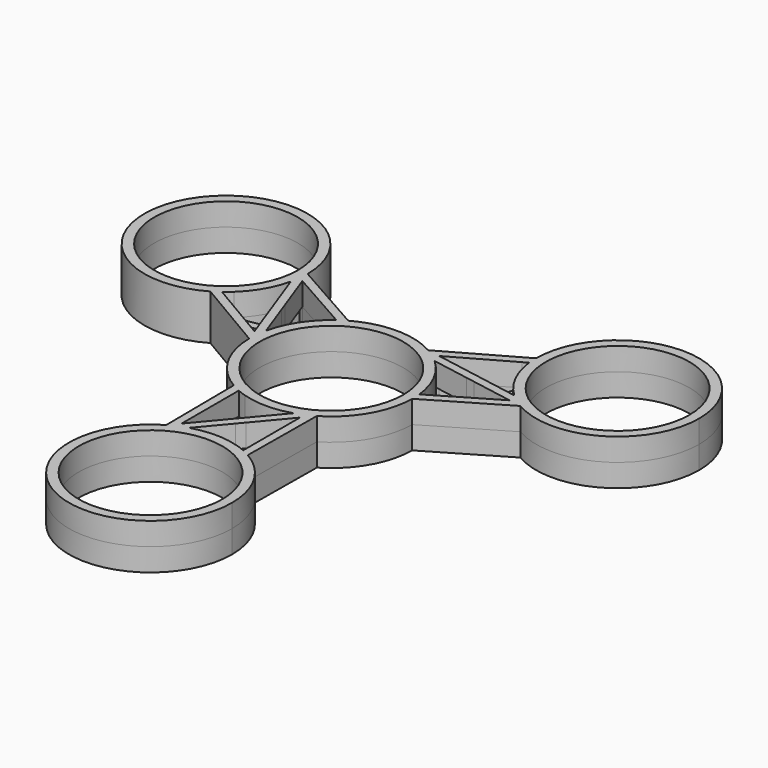
from build123d import *

# Parameters (mm, degrees)
F0_R     = 11.0625
F1_DEPTH = 3.5
F2_DEPTH = 3.5


with BuildPart() as f1:
    # F0 (on Top) → F1 (new body)
    with BuildSketch(Plane.XY):
        with BuildLine():
            ThreePointArc((12.5625, -34.825), (10.879444135, -28.54375), (6.28125, -23.945555865))
            ThreePointArc((6.28125, -23.945555865), (5.6839265838, -23.6219028907), (5.0699800766, -23.3310142565))
            ThreePointArc((5.0699800766, -23.3310142565), (4.3783795457, -23.0501879504), (3.671321038, -22.8109329082))
            ThreePointArc((3.671321038, -22.8109329082), (0, -22.2625), (-3.671321038, -22.8109329082))
            ThreePointArc((-3.671321038, -22.8109329082), (-4.3783795457, -23.0501879504), (-5.0699800766, -23.3310142565))
            ThreePointArc((-5.0699800766, -23.3310142565), (-5.6839265838, -23.6219028907), (-6.28125, -23.945555865))
            ThreePointArc((-6.28125, -23.945555865), (-6.28125, -45.704444135), (12.5625, -34.825))
        make_face()
        with Locations((0, -34.825)):
            Circle(F0_R, mode=Mode.SUBTRACT)
        with BuildLine():
            ThreePointArc((22.6934953293, 7.3091515977), (23.2748450472, 6.9043979519), (23.8780846868, 6.533055865))
            ThreePointArc((23.8780846868, 6.533055865), (36.4405846868, 6.533055865), (42.7218346868, 17.4125))
            ThreePointArc((42.7218346868, 17.4125), (30.1593346868, 29.975), (17.5968346868, 17.4125))
            ThreePointArc((17.5968346868, 17.4125), (17.6168065478, 16.7044081041), (17.6766586284, 15.998567657))
            ThreePointArc((17.6766586284, 15.998567657), (17.777731299, 15.2882816033), (17.9191868635, 14.5849237385))
            ThreePointArc((17.9191868635, 14.5849237385), (19.2798905518, 11.13125), (21.5905079016, 8.2260091697))
            ThreePointArc((21.5905079016, 8.2260091697), (22.1289058982, 7.7518261249), (22.6934953293, 7.3091515977))
        make_face()
        with Locations((30.1593346868, 17.4125)):
            Circle(F0_R, mode=Mode.SUBTRACT)
        with BuildLine():
            ThreePointArc((-17.6766586284, 15.998567657), (-17.6168065478, 16.7044081041), (-17.5968346868, 17.4125))
            ThreePointArc((-17.5968346868, 17.4125), (-41.0387788218, 23.69375), (-23.8780846868, 6.533055865))
            ThreePointArc((-23.8780846868, 6.533055865), (-23.2748450472, 6.9043979519), (-22.6934953293, 7.3091515977))
            ThreePointArc((-22.6934953293, 7.3091515977), (-22.1289058982, 7.7518261249), (-21.5905079016, 8.2260091697))
            ThreePointArc((-21.5905079016, 8.2260091697), (-19.2798905518, 11.13125), (-17.9191868635, 14.5849237385))
            ThreePointArc((-17.9191868635, 14.5849237385), (-17.777731299, 15.2882816033), (-17.6766586284, 15.998567657))
        make_face()
        with Locations((-30.1593346868, 17.4125)):
            Circle(F0_R, mode=Mode.SUBTRACT)
        with BuildLine():
            ThreePointArc((12.5617807334, -0.134428631), (12.5623201821, -0.0672152776), (12.5625, 0))
            ThreePointArc((12.5625, 0), (12.5456200156, 0.6510181823), (12.4950254251, 1.300286844))
            ThreePointArc((12.4950254251, 1.300286844), (12.3979510712, 2.0266266272), (12.2586909143, 2.7460705232))
            ThreePointArc((12.2586909143, 2.7460705232), (10.879444135, 6.28125), (8.5075122908, 9.2433024873))
            ThreePointArc((8.5075122908, 9.2433024873), (7.9540856787, 9.723627269), (7.3735941516, 10.1708660171))
            ThreePointArc((7.3735941516, 10.1708660171), (6.7801201382, 10.5757447568), (6.1644717573, 10.9460355474))
            ThreePointArc((6.1644717573, 10.9460355474), (0, 12.5625), (-6.1644717573, 10.9460355474))
            ThreePointArc((-6.1644717573, 10.9460355474), (-6.7801201382, 10.5757447568), (-7.3735941516, 10.1708660171))
            ThreePointArc((-7.3735941516, 10.1708660171), (-7.9540856787, 9.723627269), (-8.5075122908, 9.2433024873))
            ThreePointArc((-8.5075122908, 9.2433024873), (-10.879444135, 6.28125), (-12.2586909143, 2.7460705232))
            ThreePointArc((-12.2586909143, 2.7460705232), (-12.3979510712, 2.0266266272), (-12.4950254251, 1.300286844))
            ThreePointArc((-12.4950254251, 1.300286844), (-12.5489236925, 0.583883902), (-12.5617807334, -0.134428631))
            ThreePointArc((-12.5617807334, -0.134428631), (-10.879444135, -6.28125), (-6.3973089761, -10.8116069164))
            ThreePointArc((-6.3973089761, -10.8116069164), (-5.7437870583, -11.1725250718), (-5.0699800766, -11.4939857435))
            ThreePointArc((-5.0699800766, -11.4939857435), (-4.4175289857, -11.760180437), (-3.7511786235, -11.9893730105))
            ThreePointArc((-3.7511786235, -11.9893730105), (0, -12.5625), (3.7511786235, -11.9893730105))
            ThreePointArc((3.7511786235, -11.9893730105), (4.4175289857, -11.760180437), (5.0699800766, -11.4939857435))
            ThreePointArc((5.0699800766, -11.4939857435), (5.7437870583, -11.1725250718), (6.3973089761, -10.8116069164))
            ThreePointArc((6.3973089761, -10.8116069164), (10.879444135, -6.28125), (12.5617807334, -0.134428631))
        make_face()
        Circle(F0_R, mode=Mode.SUBTRACT)
        with BuildLine():
            ThreePointArc((-22.6934953293, 7.3091515977), (-23.2748450472, 6.9043979519), (-23.8780846868, 6.533055865))
            Line((-23.8780846868, 6.533055865), (-21.9525338245, 6.8725824347))
            Line((-21.9525338245, 6.8725824347), (-22.6934953293, 7.3091515977))
        make_face()
        Polygon((-23.8780846868, 6.533055865), (-12.5617807334, -0.134428631), (-13.2447523803, 1.742020547), (-21.9525338245, 6.8725824347), align=None)
        with BuildLine():
            Line((-13.2447523803, 1.742020547), (-12.5617807334, -0.134428631))
            ThreePointArc((-12.5617807334, -0.134428631), (-12.5489236925, 0.583883902), (-12.4950254251, 1.300286844))
            Line((-12.4950254251, 1.300286844), (-13.2447523803, 1.742020547))
        make_face()
        Polygon((-8.1310102377, 10.5992817546), (-6.1644717573, 10.9460355474), (-17.5968346868, 17.4125), (-16.9280978903, 15.5751607521), align=None)
        with BuildLine():
            Line((-16.9280978903, 15.5751607521), (-17.5968346868, 17.4125))
            ThreePointArc((-17.5968346868, 17.4125), (-17.6168065478, 16.7044081041), (-17.6766586284, 15.998567657))
            Line((-17.6766586284, 15.998567657), (-16.9280978903, 15.5751607521))
        make_face()
        with BuildLine():
            ThreePointArc((-7.3735941516, 10.1708660171), (-6.7801201382, 10.5757447568), (-6.1644717573, 10.9460355474))
            Line((-6.1644717573, 10.9460355474), (-8.1310102377, 10.5992817546))
            Line((-8.1310102377, 10.5992817546), (-7.3735941516, 10.1708660171))
        make_face()
        with BuildLine():
            Line((-5.0699800766, -22.5020205822), (-6.28125, -23.945555865))
            ThreePointArc((-6.28125, -23.945555865), (-5.6839265838, -23.6219028907), (-5.0699800766, -23.3310142565))
            Line((-5.0699800766, -23.3310142565), (-5.0699800766, -22.5020205822))
        make_face()
        Polygon((-6.3973089761, -10.8116069164), (-6.28125, -23.945555865), (-5.0699800766, -22.5020205822), (-5.0699800766, -12.3934559009), align=None)
        with BuildLine():
            Line((-5.0699800766, -12.3934559009), (-5.0699800766, -11.4939857435))
            ThreePointArc((-5.0699800766, -11.4939857435), (-5.7437870583, -11.1725250718), (-6.3973089761, -10.8116069164))
            Line((-6.3973089761, -10.8116069164), (-5.0699800766, -12.3934559009))
        make_face()
        with BuildLine():
            Line((5.0699800766, -12.3934559009), (6.3973089761, -10.8116069164))
            ThreePointArc((6.3973089761, -10.8116069164), (5.7437870583, -11.1725250718), (5.0699800766, -11.4939857435))
            Line((5.0699800766, -11.4939857435), (5.0699800766, -12.3934559009))
        make_face()
        Polygon((6.28125, -23.945555865), (6.3973089761, -10.8116069164), (5.0699800766, -12.3934559009), (5.0699800766, -22.5020205822), align=None)
        with BuildLine():
            ThreePointArc((5.0699800766, -23.3310142565), (5.6839265838, -23.6219028907), (6.28125, -23.945555865))
            Line((6.28125, -23.945555865), (5.0699800766, -22.5020205822))
            Line((5.0699800766, -22.5020205822), (5.0699800766, -23.3310142565))
        make_face()
        with BuildLine():
            Line((-3.671321038, -22.8109329082), (0, -18.4356228716))
            Line((0, -18.4356228716), (-0.8289336287, -17.4477382415))
            Line((-0.8289336287, -17.4477382415), (-5.0699800766, -22.5020205822))
            Line((-5.0699800766, -22.5020205822), (-5.0699800766, -23.3310142565))
            ThreePointArc((-5.0699800766, -23.3310142565), (-4.3783795457, -23.0501879504), (-3.671321038, -22.8109329082))
        make_face()
        Polygon((0, -18.4356228716), (0.8289336287, -17.4477382415), (0, -16.4598536115), (-0.8289336287, -17.4477382415), align=None)
        with BuildLine():
            Line((5.0699800766, -12.3934559009), (5.0699800766, -11.4939857435))
            ThreePointArc((5.0699800766, -11.4939857435), (4.4175289857, -11.760180437), (3.7511786235, -11.9893730105))
            Line((3.7511786235, -11.9893730105), (0, -16.4598536115))
            Line((0, -16.4598536115), (0.8289336287, -17.4477382415))
            Line((0.8289336287, -17.4477382415), (5.0699800766, -12.3934559009))
        make_face()
        Polygon((13.2447523803, 1.742020547), (12.5617807334, -0.134428631), (23.8780846868, 6.533055865), (21.9525338245, 6.8725824347), align=None)
        with BuildLine():
            ThreePointArc((12.4950254251, 1.300286844), (12.5456200156, 0.6510181823), (12.5625, 0))
            ThreePointArc((12.5625, 0), (12.5623201821, -0.0672152776), (12.5617807334, -0.134428631))
            Line((12.5617807334, -0.134428631), (13.2447523803, 1.742020547))
            Line((13.2447523803, 1.742020547), (12.4950254251, 1.300286844))
        make_face()
        with BuildLine():
            Line((21.9525338245, 6.8725824347), (23.8780846868, 6.533055865))
            ThreePointArc((23.8780846868, 6.533055865), (23.2748450472, 6.9043979519), (22.6934953293, 7.3091515977))
            Line((22.6934953293, 7.3091515977), (21.9525338245, 6.8725824347))
        make_face()
        Polygon((16.9280978903, 15.5751607521), (17.5968346868, 17.4125), (6.1644717573, 10.9460355474), (8.1310102377, 10.5992817546), align=None)
        with BuildLine():
            ThreePointArc((6.1644717573, 10.9460355474), (6.7801201382, 10.5757447568), (7.3735941516, 10.1708660171))
            Line((7.3735941516, 10.1708660171), (8.1310102377, 10.5992817546))
            Line((8.1310102377, 10.5992817546), (6.1644717573, 10.9460355474))
        make_face()
        with BuildLine():
            ThreePointArc((17.6766586284, 15.998567657), (17.6168065478, 16.7044081041), (17.5968346868, 17.4125))
            Line((17.5968346868, 17.4125), (16.9280978903, 15.5751607521))
            Line((16.9280978903, 15.5751607521), (17.6766586284, 15.998567657))
        make_face()
        with BuildLine():
            Line((15.9657177414, 9.2178114358), (15.5246513701, 8.0059915402))
            Line((15.5246513701, 8.0059915402), (21.9525338245, 6.8725824347))
            Line((21.9525338245, 6.8725824347), (22.6934953293, 7.3091515977))
            ThreePointArc((22.6934953293, 7.3091515977), (22.1289058982, 7.7518261249), (21.5905079016, 8.2260091697))
            Line((21.5905079016, 8.2260091697), (15.9657177414, 9.2178114358))
        make_face()
        Polygon((14.6957177414, 9.4417467013), (14.2546513701, 8.2299268057), (15.5246513701, 8.0059915402), (15.9657177414, 9.2178114358), align=None)
        with BuildLine():
            ThreePointArc((7.3735941516, 10.1708660171), (7.9540856787, 9.723627269), (8.5075122908, 9.2433024873))
            Line((8.5075122908, 9.2433024873), (14.2546513701, 8.2299268057))
            Line((14.2546513701, 8.2299268057), (14.6957177414, 9.4417467013))
            Line((14.6957177414, 9.4417467013), (8.1310102377, 10.5992817546))
            Line((8.1310102377, 10.5992817546), (7.3735941516, 10.1708660171))
        make_face()
        with BuildLine():
            Line((-15.9657177414, 9.2178114358), (-14.6957177414, 9.4417467013))
            Line((-14.6957177414, 9.4417467013), (-16.9280978903, 15.5751607521))
            Line((-16.9280978903, 15.5751607521), (-17.6766586284, 15.998567657))
            ThreePointArc((-17.6766586284, 15.998567657), (-17.777731299, 15.2882816033), (-17.9191868635, 14.5849237385))
            Line((-17.9191868635, 14.5849237385), (-15.9657177414, 9.2178114358))
        make_face()
        Polygon((-14.2546513701, 8.2299268057), (-14.6957177414, 9.4417467013), (-15.9657177414, 9.2178114358), (-15.5246513701, 8.0059915402), align=None)
        with BuildLine():
            Line((-13.2447523803, 1.742020547), (-12.4950254251, 1.300286844))
            ThreePointArc((-12.4950254251, 1.300286844), (-12.3979510712, 2.0266266272), (-12.2586909143, 2.7460705232))
            Line((-12.2586909143, 2.7460705232), (-14.2546513701, 8.2299268057))
            Line((-14.2546513701, 8.2299268057), (-15.5246513701, 8.0059915402))
            Line((-15.5246513701, 8.0059915402), (-13.2447523803, 1.742020547))
        make_face()
    extrude(amount=F1_DEPTH)

    # F0 (on Top) → F2 (join)
    with BuildSketch(Plane.XY):
        with BuildLine():
            Line((-13.2447523803, 1.742020547), (-12.5617807334, -0.134428631))
            ThreePointArc((-12.5617807334, -0.134428631), (-12.5489236925, 0.583883902), (-12.4950254251, 1.300286844))
            Line((-12.4950254251, 1.300286844), (-13.2447523803, 1.742020547))
        make_face()
        Polygon((-23.8780846868, 6.533055865), (-12.5617807334, -0.134428631), (-13.2447523803, 1.742020547), (-21.9525338245, 6.8725824347), align=None)
        with BuildLine():
            ThreePointArc((-22.6934953293, 7.3091515977), (-23.2748450472, 6.9043979519), (-23.8780846868, 6.533055865))
            Line((-23.8780846868, 6.533055865), (-21.9525338245, 6.8725824347))
            Line((-21.9525338245, 6.8725824347), (-22.6934953293, 7.3091515977))
        make_face()
        with BuildLine():
            ThreePointArc((-17.6766586284, 15.998567657), (-17.6168065478, 16.7044081041), (-17.5968346868, 17.4125))
            ThreePointArc((-17.5968346868, 17.4125), (-41.0387788218, 23.69375), (-23.8780846868, 6.533055865))
            ThreePointArc((-23.8780846868, 6.533055865), (-23.2748450472, 6.9043979519), (-22.6934953293, 7.3091515977))
            ThreePointArc((-22.6934953293, 7.3091515977), (-22.1289058982, 7.7518261249), (-21.5905079016, 8.2260091697))
            ThreePointArc((-21.5905079016, 8.2260091697), (-19.2798905518, 11.13125), (-17.9191868635, 14.5849237385))
            ThreePointArc((-17.9191868635, 14.5849237385), (-17.777731299, 15.2882816033), (-17.6766586284, 15.998567657))
        make_face()
        with Locations((-30.1593346868, 17.4125)):
            Circle(F0_R, mode=Mode.SUBTRACT)
        with BuildLine():
            Line((-16.9280978903, 15.5751607521), (-17.5968346868, 17.4125))
            ThreePointArc((-17.5968346868, 17.4125), (-17.6168065478, 16.7044081041), (-17.6766586284, 15.998567657))
            Line((-17.6766586284, 15.998567657), (-16.9280978903, 15.5751607521))
        make_face()
        Polygon((-8.1310102377, 10.5992817546), (-6.1644717573, 10.9460355474), (-17.5968346868, 17.4125), (-16.9280978903, 15.5751607521), align=None)
        with BuildLine():
            ThreePointArc((-7.3735941516, 10.1708660171), (-6.7801201382, 10.5757447568), (-6.1644717573, 10.9460355474))
            Line((-6.1644717573, 10.9460355474), (-8.1310102377, 10.5992817546))
            Line((-8.1310102377, 10.5992817546), (-7.3735941516, 10.1708660171))
        make_face()
        with BuildLine():
            ThreePointArc((22.6934953293, 7.3091515977), (23.2748450472, 6.9043979519), (23.8780846868, 6.533055865))
            ThreePointArc((23.8780846868, 6.533055865), (36.4405846868, 6.533055865), (42.7218346868, 17.4125))
            ThreePointArc((42.7218346868, 17.4125), (30.1593346868, 29.975), (17.5968346868, 17.4125))
            ThreePointArc((17.5968346868, 17.4125), (17.6168065478, 16.7044081041), (17.6766586284, 15.998567657))
            ThreePointArc((17.6766586284, 15.998567657), (17.777731299, 15.2882816033), (17.9191868635, 14.5849237385))
            ThreePointArc((17.9191868635, 14.5849237385), (19.2798905518, 11.13125), (21.5905079016, 8.2260091697))
            ThreePointArc((21.5905079016, 8.2260091697), (22.1289058982, 7.7518261249), (22.6934953293, 7.3091515977))
        make_face()
        with Locations((30.1593346868, 17.4125)):
            Circle(F0_R, mode=Mode.SUBTRACT)
        with BuildLine():
            ThreePointArc((17.6766586284, 15.998567657), (17.6168065478, 16.7044081041), (17.5968346868, 17.4125))
            Line((17.5968346868, 17.4125), (16.9280978903, 15.5751607521))
            Line((16.9280978903, 15.5751607521), (17.6766586284, 15.998567657))
        make_face()
        Polygon((16.9280978903, 15.5751607521), (17.5968346868, 17.4125), (6.1644717573, 10.9460355474), (8.1310102377, 10.5992817546), align=None)
        with BuildLine():
            ThreePointArc((6.1644717573, 10.9460355474), (6.7801201382, 10.5757447568), (7.3735941516, 10.1708660171))
            Line((7.3735941516, 10.1708660171), (8.1310102377, 10.5992817546))
            Line((8.1310102377, 10.5992817546), (6.1644717573, 10.9460355474))
        make_face()
        Polygon((13.2447523803, 1.742020547), (12.5617807334, -0.134428631), (23.8780846868, 6.533055865), (21.9525338245, 6.8725824347), align=None)
        with BuildLine():
            Line((21.9525338245, 6.8725824347), (23.8780846868, 6.533055865))
            ThreePointArc((23.8780846868, 6.533055865), (23.2748450472, 6.9043979519), (22.6934953293, 7.3091515977))
            Line((22.6934953293, 7.3091515977), (21.9525338245, 6.8725824347))
        make_face()
        with BuildLine():
            ThreePointArc((12.4950254251, 1.300286844), (12.5456200156, 0.6510181823), (12.5625, 0))
            ThreePointArc((12.5625, 0), (12.5623201821, -0.0672152776), (12.5617807334, -0.134428631))
            Line((12.5617807334, -0.134428631), (13.2447523803, 1.742020547))
            Line((13.2447523803, 1.742020547), (12.4950254251, 1.300286844))
        make_face()
        with BuildLine():
            ThreePointArc((12.5625, -34.825), (10.879444135, -28.54375), (6.28125, -23.945555865))
            ThreePointArc((6.28125, -23.945555865), (5.6839265838, -23.6219028907), (5.0699800766, -23.3310142565))
            ThreePointArc((5.0699800766, -23.3310142565), (4.3783795457, -23.0501879504), (3.671321038, -22.8109329082))
            ThreePointArc((3.671321038, -22.8109329082), (0, -22.2625), (-3.671321038, -22.8109329082))
            ThreePointArc((-3.671321038, -22.8109329082), (-4.3783795457, -23.0501879504), (-5.0699800766, -23.3310142565))
            ThreePointArc((-5.0699800766, -23.3310142565), (-5.6839265838, -23.6219028907), (-6.28125, -23.945555865))
            ThreePointArc((-6.28125, -23.945555865), (-6.28125, -45.704444135), (12.5625, -34.825))
        make_face()
        with Locations((0, -34.825)):
            Circle(F0_R, mode=Mode.SUBTRACT)
        with BuildLine():
            ThreePointArc((5.0699800766, -23.3310142565), (5.6839265838, -23.6219028907), (6.28125, -23.945555865))
            Line((6.28125, -23.945555865), (5.0699800766, -22.5020205822))
            Line((5.0699800766, -22.5020205822), (5.0699800766, -23.3310142565))
        make_face()
        with BuildLine():
            Line((-5.0699800766, -22.5020205822), (-6.28125, -23.945555865))
            ThreePointArc((-6.28125, -23.945555865), (-5.6839265838, -23.6219028907), (-5.0699800766, -23.3310142565))
            Line((-5.0699800766, -23.3310142565), (-5.0699800766, -22.5020205822))
        make_face()
        Polygon((-6.3973089761, -10.8116069164), (-6.28125, -23.945555865), (-5.0699800766, -22.5020205822), (-5.0699800766, -12.3934559009), align=None)
        Polygon((6.28125, -23.945555865), (6.3973089761, -10.8116069164), (5.0699800766, -12.3934559009), (5.0699800766, -22.5020205822), align=None)
        with BuildLine():
            Line((-5.0699800766, -12.3934559009), (-5.0699800766, -11.4939857435))
            ThreePointArc((-5.0699800766, -11.4939857435), (-5.7437870583, -11.1725250718), (-6.3973089761, -10.8116069164))
            Line((-6.3973089761, -10.8116069164), (-5.0699800766, -12.3934559009))
        make_face()
        with BuildLine():
            Line((5.0699800766, -12.3934559009), (6.3973089761, -10.8116069164))
            ThreePointArc((6.3973089761, -10.8116069164), (5.7437870583, -11.1725250718), (5.0699800766, -11.4939857435))
            Line((5.0699800766, -11.4939857435), (5.0699800766, -12.3934559009))
        make_face()
        with BuildLine():
            ThreePointArc((12.5617807334, -0.134428631), (12.5623201821, -0.0672152776), (12.5625, 0))
            ThreePointArc((12.5625, 0), (12.5456200156, 0.6510181823), (12.4950254251, 1.300286844))
            ThreePointArc((12.4950254251, 1.300286844), (12.3979510712, 2.0266266272), (12.2586909143, 2.7460705232))
            ThreePointArc((12.2586909143, 2.7460705232), (10.879444135, 6.28125), (8.5075122908, 9.2433024873))
            ThreePointArc((8.5075122908, 9.2433024873), (7.9540856787, 9.723627269), (7.3735941516, 10.1708660171))
            ThreePointArc((7.3735941516, 10.1708660171), (6.7801201382, 10.5757447568), (6.1644717573, 10.9460355474))
            ThreePointArc((6.1644717573, 10.9460355474), (0, 12.5625), (-6.1644717573, 10.9460355474))
            ThreePointArc((-6.1644717573, 10.9460355474), (-6.7801201382, 10.5757447568), (-7.3735941516, 10.1708660171))
            ThreePointArc((-7.3735941516, 10.1708660171), (-7.9540856787, 9.723627269), (-8.5075122908, 9.2433024873))
            ThreePointArc((-8.5075122908, 9.2433024873), (-10.879444135, 6.28125), (-12.2586909143, 2.7460705232))
            ThreePointArc((-12.2586909143, 2.7460705232), (-12.3979510712, 2.0266266272), (-12.4950254251, 1.300286844))
            ThreePointArc((-12.4950254251, 1.300286844), (-12.5489236925, 0.583883902), (-12.5617807334, -0.134428631))
            ThreePointArc((-12.5617807334, -0.134428631), (-10.879444135, -6.28125), (-6.3973089761, -10.8116069164))
            ThreePointArc((-6.3973089761, -10.8116069164), (-5.7437870583, -11.1725250718), (-5.0699800766, -11.4939857435))
            ThreePointArc((-5.0699800766, -11.4939857435), (-4.4175289857, -11.760180437), (-3.7511786235, -11.9893730105))
            ThreePointArc((-3.7511786235, -11.9893730105), (0, -12.5625), (3.7511786235, -11.9893730105))
            ThreePointArc((3.7511786235, -11.9893730105), (4.4175289857, -11.760180437), (5.0699800766, -11.4939857435))
            ThreePointArc((5.0699800766, -11.4939857435), (5.7437870583, -11.1725250718), (6.3973089761, -10.8116069164))
            ThreePointArc((6.3973089761, -10.8116069164), (10.879444135, -6.28125), (12.5617807334, -0.134428631))
        make_face()
        Circle(F0_R, mode=Mode.SUBTRACT)
        with BuildLine():
            Line((5.0699800766, -22.5020205822), (0.8289336287, -17.4477382415))
            Line((0.8289336287, -17.4477382415), (0, -18.4356228716))
            Line((0, -18.4356228716), (3.671321038, -22.8109329082))
            ThreePointArc((3.671321038, -22.8109329082), (4.3783795457, -23.0501879504), (5.0699800766, -23.3310142565))
            Line((5.0699800766, -23.3310142565), (5.0699800766, -22.5020205822))
        make_face()
        Polygon((0, -18.4356228716), (0.8289336287, -17.4477382415), (0, -16.4598536115), (-0.8289336287, -17.4477382415), align=None)
        with BuildLine():
            Line((0, -16.4598536115), (-3.7511786235, -11.9893730105))
            ThreePointArc((-3.7511786235, -11.9893730105), (-4.4175289857, -11.760180437), (-5.0699800766, -11.4939857435))
            Line((-5.0699800766, -11.4939857435), (-5.0699800766, -12.3934559009))
            Line((-5.0699800766, -12.3934559009), (-0.8289336287, -17.4477382415))
            Line((-0.8289336287, -17.4477382415), (0, -16.4598536115))
        make_face()
        with BuildLine():
            Line((16.9280978903, 15.5751607521), (14.6957177414, 9.4417467013))
            Line((14.6957177414, 9.4417467013), (15.9657177414, 9.2178114358))
            Line((15.9657177414, 9.2178114358), (17.9191868635, 14.5849237385))
            ThreePointArc((17.9191868635, 14.5849237385), (17.777731299, 15.2882816033), (17.6766586284, 15.998567657))
            Line((17.6766586284, 15.998567657), (16.9280978903, 15.5751607521))
        make_face()
        Polygon((14.6957177414, 9.4417467013), (14.2546513701, 8.2299268057), (15.5246513701, 8.0059915402), (15.9657177414, 9.2178114358), align=None)
        with BuildLine():
            ThreePointArc((12.2586909143, 2.7460705232), (12.3979510712, 2.0266266272), (12.4950254251, 1.300286844))
            Line((12.4950254251, 1.300286844), (13.2447523803, 1.742020547))
            Line((13.2447523803, 1.742020547), (15.5246513701, 8.0059915402))
            Line((15.5246513701, 8.0059915402), (14.2546513701, 8.2299268057))
            Line((14.2546513701, 8.2299268057), (12.2586909143, 2.7460705232))
        make_face()
        with BuildLine():
            Line((-15.5246513701, 8.0059915402), (-15.9657177414, 9.2178114358))
            Line((-15.9657177414, 9.2178114358), (-21.5905079016, 8.2260091697))
            ThreePointArc((-21.5905079016, 8.2260091697), (-22.1289058982, 7.7518261249), (-22.6934953293, 7.3091515977))
            Line((-22.6934953293, 7.3091515977), (-21.9525338245, 6.8725824347))
            Line((-21.9525338245, 6.8725824347), (-15.5246513701, 8.0059915402))
        make_face()
        Polygon((-14.2546513701, 8.2299268057), (-14.6957177414, 9.4417467013), (-15.9657177414, 9.2178114358), (-15.5246513701, 8.0059915402), align=None)
        with BuildLine():
            ThreePointArc((-8.5075122908, 9.2433024873), (-7.9540856787, 9.723627269), (-7.3735941516, 10.1708660171))
            Line((-7.3735941516, 10.1708660171), (-8.1310102377, 10.5992817546))
            Line((-8.1310102377, 10.5992817546), (-14.6957177414, 9.4417467013))
            Line((-14.6957177414, 9.4417467013), (-14.2546513701, 8.2299268057))
            Line((-14.2546513701, 8.2299268057), (-8.5075122908, 9.2433024873))
        make_face()
    extrude(amount=-F2_DEPTH)


solid = f1.part
